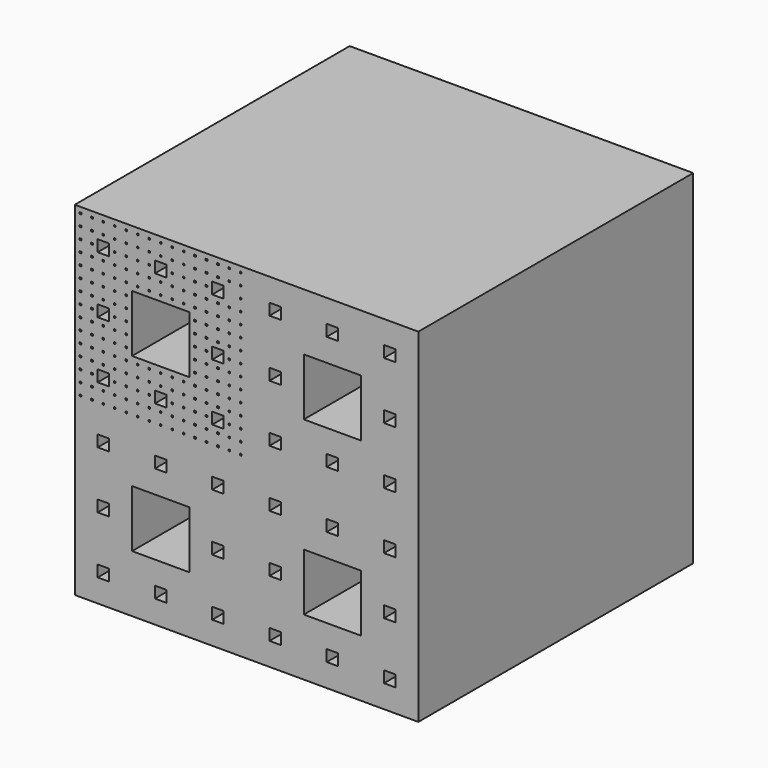
from build123d import *

# Parameters (mm, degrees)
F0_W     = 228.6
F0_H     = 228.6
F1_DEPTH = 114.3
F2_W     = 38.1
F2_H     = 38.1
F2_W_2   = 7.62
F2_H_2   = 7.62
F3_DEPTH = 228.6
F4_W     = 1.0885714286
F4_H     = 1.0885714286
F5_DEPTH = 228.6


# Not quite as in the source:
# - a feature names something its author has since deleted; it is built from what else it names


with BuildPart() as f1:
    # F0 (on Front) → F1 (new body, symmetric)
    with BuildSketch(Plane.XZ):
        Rectangle(F0_W, F0_H)
    extrude(amount=F1_DEPTH, both=True)

    # F2 (on face) → F3 (cut)
    with BuildSketch(Plane.XZ.offset(114.3)):
        with Locations((-57.15, 57.15)):
            Rectangle(F2_W, F2_H)
        with Locations((-95.25, 95.25)):
            Rectangle(F2_W_2, F2_H_2)
        with Locations((-95.25, 57.15)):
            Rectangle(F2_W_2, F2_H_2)
        with Locations((-95.25, 19.05)):
            Rectangle(F2_W_2, F2_H_2)
        with Locations((-57.15, 95.25)):
            Rectangle(F2_W_2, F2_H_2)
        with Locations((-57.15, 19.05)):
            Rectangle(F2_W_2, F2_H_2)
        with Locations((-19.05, 95.25)):
            Rectangle(F2_W_2, F2_H_2)
        with Locations((-19.05, 57.15)):
            Rectangle(F2_W_2, F2_H_2)
        with Locations((-19.05, 19.05)):
            Rectangle(F2_W_2, F2_H_2)
        with Locations((-57.15, -57.15)):
            Rectangle(F2_W, F2_H)
        with Locations((-95.25, -19.05)):
            Rectangle(F2_W_2, F2_H_2)
        with Locations((-95.25, -95.25)):
            Rectangle(F2_W_2, F2_H_2)
        with Locations((-19.05, -57.15)):
            Rectangle(F2_W_2, F2_H_2)
        with Locations((-19.05, -19.05)):
            Rectangle(F2_W_2, F2_H_2)
        with Locations((-95.25, -57.15)):
            Rectangle(F2_W_2, F2_H_2)
        with Locations((-57.15, -95.25)):
            Rectangle(F2_W_2, F2_H_2)
        with Locations((-19.05, -95.25)):
            Rectangle(F2_W_2, F2_H_2)
        with Locations((-57.15, -19.05)):
            Rectangle(F2_W_2, F2_H_2)
        with Locations((57.15, 57.15)):
            Rectangle(F2_W, F2_H)
        with Locations((19.05, 95.25)):
            Rectangle(F2_W_2, F2_H_2)
        with Locations((19.05, 19.05)):
            Rectangle(F2_W_2, F2_H_2)
        with Locations((95.25, 57.15)):
            Rectangle(F2_W_2, F2_H_2)
        with Locations((95.25, 95.25)):
            Rectangle(F2_W_2, F2_H_2)
        with Locations((19.05, 57.15)):
            Rectangle(F2_W_2, F2_H_2)
        with Locations((57.15, 19.05)):
            Rectangle(F2_W_2, F2_H_2)
        with Locations((95.25, 19.05)):
            Rectangle(F2_W_2, F2_H_2)
        with Locations((57.15, 95.25)):
            Rectangle(F2_W_2, F2_H_2)
        with Locations((57.15, -57.15)):
            Rectangle(F2_W, F2_H)
        with Locations((19.05, -19.05)):
            Rectangle(F2_W_2, F2_H_2)
        with Locations((19.05, -95.25)):
            Rectangle(F2_W_2, F2_H_2)
        with Locations((95.25, -57.15)):
            Rectangle(F2_W_2, F2_H_2)
        with Locations((95.25, -19.05)):
            Rectangle(F2_W_2, F2_H_2)
        with Locations((19.05, -57.15)):
            Rectangle(F2_W_2, F2_H_2)
        with Locations((57.15, -95.25)):
            Rectangle(F2_W_2, F2_H_2)
        with Locations((95.25, -95.25)):
            Rectangle(F2_W_2, F2_H_2)
        with Locations((57.15, -19.05)):
            Rectangle(F2_W_2, F2_H_2)
    extrude(amount=-F3_DEPTH, mode=Mode.SUBTRACT)

    # F4 (on face) → F5 (cut)
    with BuildSketch(Plane.XZ.offset(114.3)):
        with Locations((-110.49, 49.53)):
            Rectangle(F4_W, F4_H)
        with Locations((-110.49, 41.91)):
            Rectangle(F4_W, F4_H)
        with Locations((-110.49, 64.77)):
            Rectangle(F4_W, F4_H)
        with Locations((-110.49, 57.15)):
            Rectangle(F4_W, F4_H)
        with Locations((-110.49, 72.39)):
            Rectangle(F4_W, F4_H)
        with Locations((-80.01, 3.81)):
            Rectangle(F4_W, F4_H)
        with Locations((-95.25, 3.81)):
            Rectangle(F4_W, F4_H)
        with Locations((-102.87, 3.81)):
            Rectangle(F4_W, F4_H)
        with Locations((-110.49, 11.43)):
            Rectangle(F4_W, F4_H)
        with Locations((-110.49, 3.81)):
            Rectangle(F4_W, F4_H)
        with Locations((-110.49, 26.67)):
            Rectangle(F4_W, F4_H)
        with Locations((-110.49, 19.05)):
            Rectangle(F4_W, F4_H)
        with Locations((-87.63, 3.81)):
            Rectangle(F4_W, F4_H)
        with Locations((-110.49, 34.29)):
            Rectangle(F4_W, F4_H)
        with Locations((-64.77, 110.49)):
            Rectangle(F4_W, F4_H)
        with Locations((-49.53, 110.49)):
            Rectangle(F4_W, F4_H)
        with Locations((-57.15, 110.49)):
            Rectangle(F4_W, F4_H)
        with Locations((-41.91, 110.49)):
            Rectangle(F4_W, F4_H)
        with Locations((-72.39, 110.49)):
            Rectangle(F4_W, F4_H)
        with Locations((-41.91, 3.81)):
            Rectangle(F4_W, F4_H)
        with Locations((-57.15, 3.81)):
            Rectangle(F4_W, F4_H)
        with Locations((-64.77, 3.81)):
            Rectangle(F4_W, F4_H)
        with Locations((-72.39, 3.81)):
            Rectangle(F4_W, F4_H)
        with Locations((-49.53, 3.81)):
            Rectangle(F4_W, F4_H)
        with Locations((-3.81, 80.01)):
            Rectangle(F4_W, F4_H)
        with Locations((-26.67, 110.49)):
            Rectangle(F4_W, F4_H)
        with Locations((-3.81, 102.87)):
            Rectangle(F4_W, F4_H)
        with Locations((-3.81, 87.63)):
            Rectangle(F4_W, F4_H)
        with Locations((-3.81, 95.25)):
            Rectangle(F4_W, F4_H)
        with Locations((-11.43, 110.49)):
            Rectangle(F4_W, F4_H)
        with Locations((-19.05, 110.49)):
            Rectangle(F4_W, F4_H)
        with Locations((-3.81, 110.49)):
            Rectangle(F4_W, F4_H)
        with Locations((-34.29, 110.49)):
            Rectangle(F4_W, F4_H)
        with Locations((-3.81, 41.91)):
            Rectangle(F4_W, F4_H)
        with Locations((-3.81, 64.77)):
            Rectangle(F4_W, F4_H)
        with Locations((-3.81, 49.53)):
            Rectangle(F4_W, F4_H)
        with Locations((-3.81, 57.15)):
            Rectangle(F4_W, F4_H)
        with Locations((-3.81, 72.39)):
            Rectangle(F4_W, F4_H)
        with Locations((-3.81, 3.81)):
            Rectangle(F4_W, F4_H)
        with Locations((-19.05, 3.81)):
            Rectangle(F4_W, F4_H)
        with Locations((-26.67, 3.81)):
            Rectangle(F4_W, F4_H)
        with Locations((-3.81, 26.67)):
            Rectangle(F4_W, F4_H)
        with Locations((-34.29, 3.81)):
            Rectangle(F4_W, F4_H)
        with Locations((-11.43, 3.81)):
            Rectangle(F4_W, F4_H)
        with Locations((-3.81, 11.43)):
            Rectangle(F4_W, F4_H)
        with Locations((-3.81, 19.05)):
            Rectangle(F4_W, F4_H)
        with Locations((-3.81, 34.29)):
            Rectangle(F4_W, F4_H)
        with Locations((-87.63, 110.49)):
            Rectangle(F4_W, F4_H)
        with Locations((-95.25, 110.49)):
            Rectangle(F4_W, F4_H)
        with Locations((-102.87, 110.49)):
            Rectangle(F4_W, F4_H)
        with Locations((-110.49, 110.49)):
            Rectangle(F4_W, F4_H)
        with Locations((-102.87, 102.87)):
            Rectangle(F4_W, F4_H)
        with Locations((-95.25, 102.87)):
            Rectangle(F4_W, F4_H)
        with Locations((-87.63, 102.87)):
            Rectangle(F4_W, F4_H)
        with Locations((-80.01, 102.87)):
            Rectangle(F4_W, F4_H)
        with Locations((-80.01, 110.49)):
            Rectangle(F4_W, F4_H)
        with Locations((-72.39, 102.87)):
            Rectangle(F4_W, F4_H)
        with Locations((-110.49, 95.25)):
            Rectangle(F4_W, F4_H)
        with Locations((-102.87, 95.25)):
            Rectangle(F4_W, F4_H)
        with Locations((-87.63, 95.25)):
            Rectangle(F4_W, F4_H)
        with Locations((-80.01, 95.25)):
            Rectangle(F4_W, F4_H)
        with Locations((-72.39, 95.25)):
            Rectangle(F4_W, F4_H)
        with Locations((-110.49, 102.87)):
            Rectangle(F4_W, F4_H)
        with Locations((-64.77, 102.87)):
            Rectangle(F4_W, F4_H)
        with Locations((-64.77, 95.25)):
            Rectangle(F4_W, F4_H)
        with Locations((-64.77, 87.63)):
            Rectangle(F4_W, F4_H)
        with Locations((-72.39, 87.63)):
            Rectangle(F4_W, F4_H)
        with Locations((-80.01, 87.63)):
            Rectangle(F4_W, F4_H)
        with Locations((-87.63, 87.63)):
            Rectangle(F4_W, F4_H)
        with Locations((-95.25, 87.63)):
            Rectangle(F4_W, F4_H)
        with Locations((-102.87, 87.63)):
            Rectangle(F4_W, F4_H)
        with Locations((-110.49, 87.63)):
            Rectangle(F4_W, F4_H)
        with Locations((-110.49, 80.01)):
            Rectangle(F4_W, F4_H)
        with Locations((-102.87, 80.01)):
            Rectangle(F4_W, F4_H)
        with Locations((-95.25, 80.01)):
            Rectangle(F4_W, F4_H)
        with Locations((-80.01, 80.01)):
            Rectangle(F4_W, F4_H)
        with Locations((-72.39, 80.01)):
            Rectangle(F4_W, F4_H)
        with Locations((-64.77, 80.01)):
            Rectangle(F4_W, F4_H)
        with Locations((-57.15, 80.01)):
            Rectangle(F4_W, F4_H)
        with Locations((-102.87, 64.77)):
            Rectangle(F4_W, F4_H)
        with Locations((-95.25, 64.77)):
            Rectangle(F4_W, F4_H)
        with Locations((-95.25, 72.39)):
            Rectangle(F4_W, F4_H)
        with Locations((-102.87, 72.39)):
            Rectangle(F4_W, F4_H)
        with Locations((-87.63, 72.39)):
            Rectangle(F4_W, F4_H)
        with Locations((-87.63, 80.01)):
            Rectangle(F4_W, F4_H)
        with Locations((-80.01, 72.39)):
            Rectangle(F4_W, F4_H)
        with Locations((-80.01, 64.77)):
            Rectangle(F4_W, F4_H)
        with Locations((-80.01, 57.15)):
            Rectangle(F4_W, F4_H)
        with Locations((-80.01, 49.53)):
            Rectangle(F4_W, F4_H)
        with Locations((-87.63, 49.53)):
            Rectangle(F4_W, F4_H)
        with Locations((-87.63, 57.15)):
            Rectangle(F4_W, F4_H)
        with Locations((-95.25, 49.53)):
            Rectangle(F4_W, F4_H)
        with Locations((-102.87, 49.53)):
            Rectangle(F4_W, F4_H)
        with Locations((-102.87, 57.15)):
            Rectangle(F4_W, F4_H)
        with Locations((-102.87, 41.91)):
            Rectangle(F4_W, F4_H)
        with Locations((-95.25, 41.91)):
            Rectangle(F4_W, F4_H)
        with Locations((-87.63, 41.91)):
            Rectangle(F4_W, F4_H)
        with Locations((-80.01, 41.91)):
            Rectangle(F4_W, F4_H)
        with Locations((-87.63, 64.77)):
            Rectangle(F4_W, F4_H)
        with Locations((-102.87, 34.29)):
            Rectangle(F4_W, F4_H)
        with Locations((-95.25, 34.29)):
            Rectangle(F4_W, F4_H)
        with Locations((-87.63, 34.29)):
            Rectangle(F4_W, F4_H)
        with Locations((-80.01, 34.29)):
            Rectangle(F4_W, F4_H)
        with Locations((-72.39, 34.29)):
            Rectangle(F4_W, F4_H)
        with Locations((-64.77, 34.29)):
            Rectangle(F4_W, F4_H)
        with Locations((-102.87, 26.67)):
            Rectangle(F4_W, F4_H)
        with Locations((-95.25, 26.67)):
            Rectangle(F4_W, F4_H)
        with Locations((-87.63, 26.67)):
            Rectangle(F4_W, F4_H)
        with Locations((-80.01, 26.67)):
            Rectangle(F4_W, F4_H)
        with Locations((-72.39, 26.67)):
            Rectangle(F4_W, F4_H)
        with Locations((-64.77, 26.67)):
            Rectangle(F4_W, F4_H)
        with Locations((-87.63, 19.05)):
            Rectangle(F4_W, F4_H)
        with Locations((-80.01, 19.05)):
            Rectangle(F4_W, F4_H)
        with Locations((-72.39, 19.05)):
            Rectangle(F4_W, F4_H)
        with Locations((-64.77, 19.05)):
            Rectangle(F4_W, F4_H)
        with Locations((-102.87, 19.05)):
            Rectangle(F4_W, F4_H)
        with Locations((-102.87, 11.43)):
            Rectangle(F4_W, F4_H)
        with Locations((-95.25, 11.43)):
            Rectangle(F4_W, F4_H)
        with Locations((-87.63, 11.43)):
            Rectangle(F4_W, F4_H)
        with Locations((-72.39, 11.43)):
            Rectangle(F4_W, F4_H)
        with Locations((-80.01, 11.43)):
            Rectangle(F4_W, F4_H)
        with Locations((-64.77, 11.43)):
            Rectangle(F4_W, F4_H)
        with Locations((-57.15, 11.43)):
            Rectangle(F4_W, F4_H)
        with Locations((-49.53, 11.43)):
            Rectangle(F4_W, F4_H)
        with Locations((-49.53, 19.05)):
            Rectangle(F4_W, F4_H)
        with Locations((-41.91, 19.05)):
            Rectangle(F4_W, F4_H)
        with Locations((-41.91, 26.67)):
            Rectangle(F4_W, F4_H)
        with Locations((-41.91, 34.29)):
            Rectangle(F4_W, F4_H)
        with Locations((-49.53, 34.29)):
            Rectangle(F4_W, F4_H)
        with Locations((-57.15, 34.29)):
            Rectangle(F4_W, F4_H)
        with Locations((-57.15, 26.67)):
            Rectangle(F4_W, F4_H)
        with Locations((-49.53, 26.67)):
            Rectangle(F4_W, F4_H)
        with Locations((-41.91, 11.43)):
            Rectangle(F4_W, F4_H)
        with Locations((-34.29, 11.43)):
            Rectangle(F4_W, F4_H)
        with Locations((-34.29, 19.05)):
            Rectangle(F4_W, F4_H)
        with Locations((-34.29, 26.67)):
            Rectangle(F4_W, F4_H)
        with Locations((-26.67, 26.67)):
            Rectangle(F4_W, F4_H)
        with Locations((-19.05, 11.43)):
            Rectangle(F4_W, F4_H)
        with Locations((-11.43, 19.05)):
            Rectangle(F4_W, F4_H)
        with Locations((-11.43, 26.67)):
            Rectangle(F4_W, F4_H)
        with Locations((-19.05, 26.67)):
            Rectangle(F4_W, F4_H)
        with Locations((-26.67, 19.05)):
            Rectangle(F4_W, F4_H)
        with Locations((-26.67, 11.43)):
            Rectangle(F4_W, F4_H)
        with Locations((-11.43, 11.43)):
            Rectangle(F4_W, F4_H)
        with Locations((-11.43, 34.29)):
            Rectangle(F4_W, F4_H)
        with Locations((-19.05, 34.29)):
            Rectangle(F4_W, F4_H)
        with Locations((-26.67, 34.29)):
            Rectangle(F4_W, F4_H)
        with Locations((-34.29, 34.29)):
            Rectangle(F4_W, F4_H)
        with Locations((-34.29, 41.91)):
            Rectangle(F4_W, F4_H)
        with Locations((-26.67, 41.91)):
            Rectangle(F4_W, F4_H)
        with Locations((-19.05, 41.91)):
            Rectangle(F4_W, F4_H)
        with Locations((-11.43, 41.91)):
            Rectangle(F4_W, F4_H)
        with Locations((-26.67, 49.53)):
            Rectangle(F4_W, F4_H)
        with Locations((-34.29, 49.53)):
            Rectangle(F4_W, F4_H)
        with Locations((-34.29, 57.15)):
            Rectangle(F4_W, F4_H)
        with Locations((-34.29, 64.77)):
            Rectangle(F4_W, F4_H)
        with Locations((-26.67, 64.77)):
            Rectangle(F4_W, F4_H)
        with Locations((-26.67, 57.15)):
            Rectangle(F4_W, F4_H)
        with Locations((-19.05, 64.77)):
            Rectangle(F4_W, F4_H)
        with Locations((-11.43, 64.77)):
            Rectangle(F4_W, F4_H)
        with Locations((-11.43, 49.53)):
            Rectangle(F4_W, F4_H)
        with Locations((-19.05, 49.53)):
            Rectangle(F4_W, F4_H)
        with Locations((-11.43, 57.15)):
            Rectangle(F4_W, F4_H)
        with Locations((-11.43, 72.39)):
            Rectangle(F4_W, F4_H)
        with Locations((-11.43, 80.01)):
            Rectangle(F4_W, F4_H)
        with Locations((-19.05, 80.01)):
            Rectangle(F4_W, F4_H)
        with Locations((-26.67, 72.39)):
            Rectangle(F4_W, F4_H)
        with Locations((-34.29, 72.39)):
            Rectangle(F4_W, F4_H)
        with Locations((-34.29, 80.01)):
            Rectangle(F4_W, F4_H)
        with Locations((-26.67, 80.01)):
            Rectangle(F4_W, F4_H)
        with Locations((-26.67, 87.63)):
            Rectangle(F4_W, F4_H)
        with Locations((-34.29, 87.63)):
            Rectangle(F4_W, F4_H)
        with Locations((-34.29, 95.25)):
            Rectangle(F4_W, F4_H)
        with Locations((-41.91, 95.25)):
            Rectangle(F4_W, F4_H)
        with Locations((-41.91, 87.63)):
            Rectangle(F4_W, F4_H)
        with Locations((-41.91, 80.01)):
            Rectangle(F4_W, F4_H)
        with Locations((-49.53, 80.01)):
            Rectangle(F4_W, F4_H)
        with Locations((-49.53, 87.63)):
            Rectangle(F4_W, F4_H)
        with Locations((-11.43, 102.87)):
            Rectangle(F4_W, F4_H)
        with Locations((-19.05, 102.87)):
            Rectangle(F4_W, F4_H)
        with Locations((-26.67, 102.87)):
            Rectangle(F4_W, F4_H)
        with Locations((-26.67, 95.25)):
            Rectangle(F4_W, F4_H)
        with Locations((-34.29, 102.87)):
            Rectangle(F4_W, F4_H)
        with Locations((-41.91, 102.87)):
            Rectangle(F4_W, F4_H)
        with Locations((-57.15, 102.87)):
            Rectangle(F4_W, F4_H)
        with Locations((-49.53, 95.25)):
            Rectangle(F4_W, F4_H)
        with Locations((-57.15, 87.63)):
            Rectangle(F4_W, F4_H)
        with Locations((-19.05, 72.39)):
            Rectangle(F4_W, F4_H)
        with Locations((-49.53, 102.87)):
            Rectangle(F4_W, F4_H)
        with Locations((-19.05, 87.63)):
            Rectangle(F4_W, F4_H)
        with Locations((-11.43, 87.63)):
            Rectangle(F4_W, F4_H)
    extrude(amount=-F5_DEPTH, mode=Mode.SUBTRACT)


solid = f1.part
